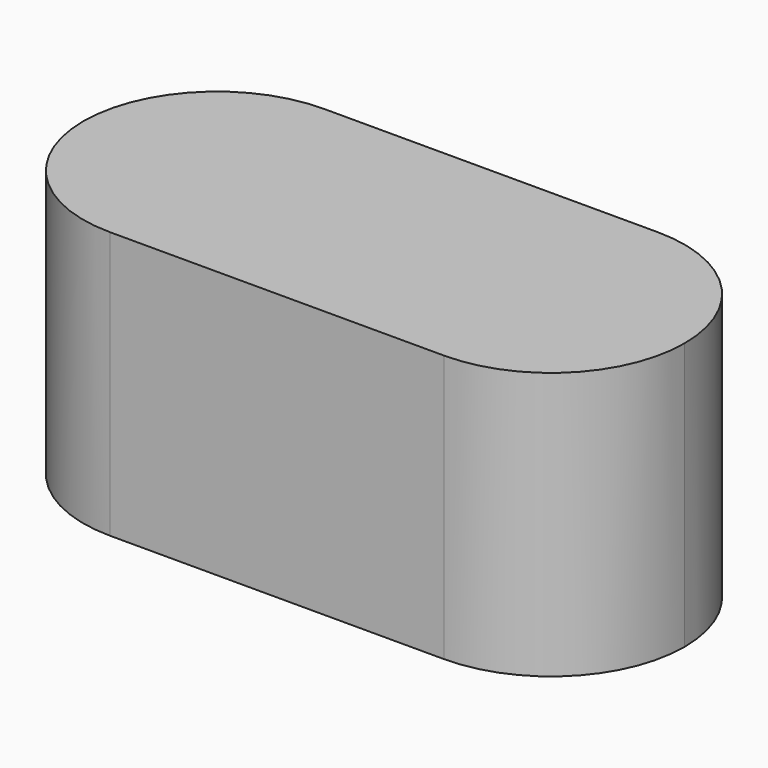
from build123d import *

# Parameters (mm, degrees)
F0_W     = 45
F0_H     = 20
F1_DEPTH = 20
F3_DEPTH = 18
F4_R     = 9.99999


# Not quite as in the source:
# - a fillet or chamfer is up to 0.001 mm smaller than in the source, because OpenCascade refuses the exact size


with BuildPart() as f1:
    # F0 (on Top) → F1 (new body)
    with BuildSketch(Plane.XY):
        Rectangle(F0_W, F0_H)
    extrude(amount=F1_DEPTH)

    # F2 (on face) → F3 (cut)
    with BuildSketch(Plane(origin=(0, 0, 0), x_dir=(1, 0, 0), z_dir=(0, 0, -1))):
        Polygon((2.6396454307, -4.572), (5.2792908615, 0), (2.6396454307, 4.572), (-2.6396454307, 4.572), (-5.2792908615, 0), (-2.6396454307, -4.572), align=None)
    extrude(amount=-F3_DEPTH, mode=Mode.SUBTRACT)

    # F4 (radius 10 in the source; OpenCascade refuses exactly that, so slightly less here)
    f4_edges = [f1.edges().sort_by_distance(p)[0] for p in [
        (22.5, -10, 10),
        (-22.5, -10, 10),
        (22.5, 10, 10),
        (-22.5, 10, 10),
    ]]
    fillet(f4_edges, radius=F4_R)


solid = f1.part
